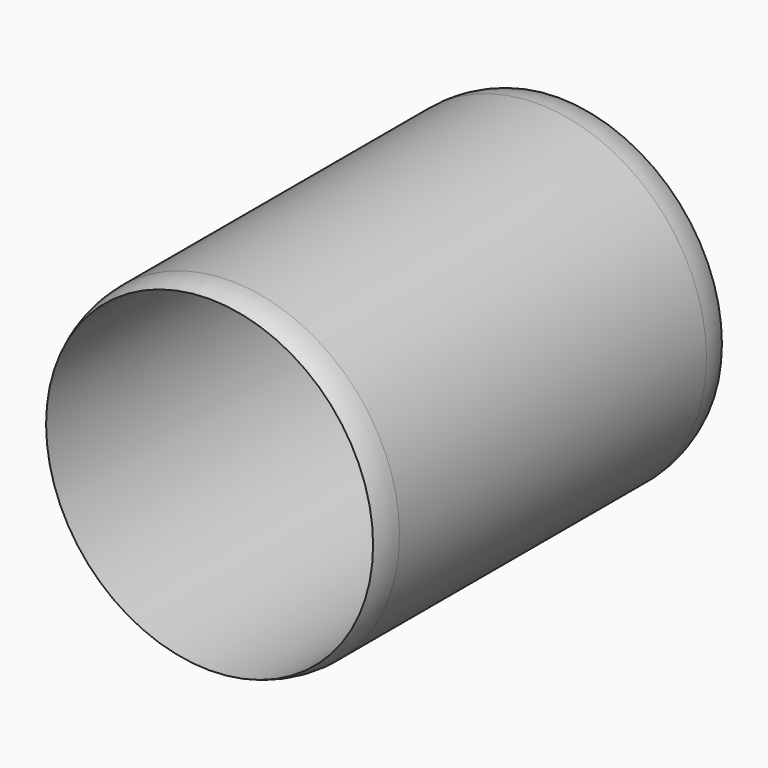
from build123d import *

# Parameters (mm, degrees)
F0_R     = 15.5
F1_DEPTH = 40
F2_R     = 15
F3_DEPTH = 40


# Not quite as in the source:
# - a fillet or chamfer that OpenCascade refuses, or shapes differently, is made with other operations: its cross-section is extruded or revolved along the edge and cut away or added


with BuildPart() as f1:
    # F0 (on Front) → F1 (new body)
    with BuildSketch(Plane.XZ):
        Circle(F0_R)
    extrude(amount=F1_DEPTH)

    # F2 (on face) → F3 (cut)
    with BuildSketch(Plane.XZ.offset(40)):
        Circle(F2_R)
    extrude(amount=-F3_DEPTH, mode=Mode.SUBTRACT)

    # F4: fillet of radius 6 on 1 edges, made by hand

    # F4_s1 → F4_t2 (revolve, cut)
    with BuildSketch(Plane.XY):
        with BuildLine():
            ThreePointArc((15.5, -37.6020842383), (15.3736700622, -38.8268291097), (15, -40))
            Line((15, -40), (15.5, -40))
            Line((15.5, -40), (15.5, -37.6020842383))
        make_face()
    revolve(axis=Axis((0, -40, 0), (0, -1, 0)), mode=Mode.SUBTRACT)

    # F5: fillet of radius 6 on 1 edges, made by hand

    # F5_s1 → F5_t2 (revolve, cut)
    with BuildSketch(Plane.XY):
        with BuildLine():
            ThreePointArc((15.5, -2.3979157617), (15.3736700622, -1.1731708903), (15, 0))
            Line((15, 0), (15.5, 0))
            Line((15.5, 0), (15.5, -2.3979157617))
        make_face()
    revolve(axis=Axis((0, 0, 0), (0, -1, 0)), mode=Mode.SUBTRACT)


solid = f1.part
